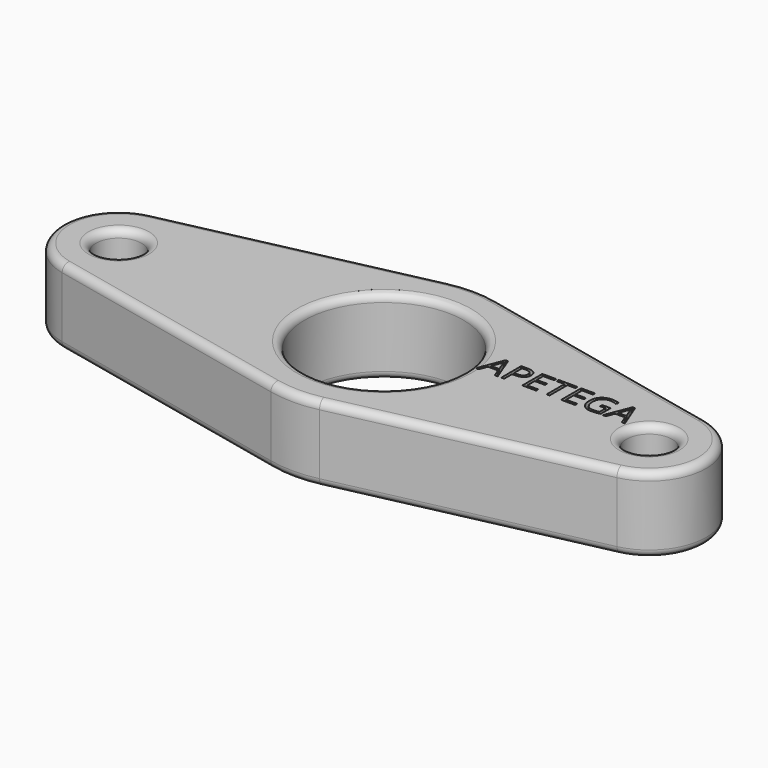
from build123d import *

# Parameters (mm, degrees)
F0_R         = 3
F0_R_2       = 10.5
F1_DEPTH     = 10
F2_R         = 1
F3_R         = 1
F4_TEXT_SIZE = 4.6232753016
F5_DEPTH     = 5


# Not quite as in the source:
# - Text() gives the source's letters only with a copy of the font that has no kerning and outlines rounded to 1/6400 em; it was checked with that copy


with BuildPart() as f1:
    # F0 (on Top) → F1 (new body)
    with BuildSketch(Plane.XY):
        with BuildLine():
            Line((-36.6071428571, -7.3257826774), (-3.2142857143, -14.6515653548))
            ThreePointArc((-3.2142857143, -14.6515653548), (0, -15), (3.2142857143, -14.6515653548))
            Line((3.2142857143, -14.6515653548), (36.6071428571, -7.3257826774))
            ThreePointArc((36.6071428571, -7.3257826774), (42.5, 0), (36.6071428571, 7.3257826774))
            Line((36.6071428571, 7.3257826774), (3.2142857143, 14.6515653548))
            ThreePointArc((3.2142857143, 14.6515653548), (0, 15), (-3.2142857143, 14.6515653548))
            Line((-3.2142857143, 14.6515653548), (-36.6071428571, 7.3257826774))
            ThreePointArc((-36.6071428571, 7.3257826774), (-42.5, 0), (-36.6071428571, -7.3257826774))
        make_face()
        with Locations((-35, 0)):
            Circle(F0_R, mode=Mode.SUBTRACT)
        Circle(F0_R_2, mode=Mode.SUBTRACT)
        with Locations((35, 0)):
            Circle(F0_R, mode=Mode.SUBTRACT)
    extrude(amount=F1_DEPTH)

    # F2
    f2_edges = [f1.edges().sort_by_distance(p)[0] for p in [
        (-19.910714, -10.988674, 10),
        (0, -15, 10),
        (19.910714, -10.988674, 10),
        (42.5, 0, 10),
        (19.910714, 10.988674, 10),
        (0, 15, 10),
        (-19.910714, 10.988674, 10),
        (-42.5, 0, 10),
        (-38, 0, 10),
        (-10.5, 0, 10),
        (32, 0, 10),
    ]]
    fillet(f2_edges, radius=F2_R)

    # F3
    f3_edges = [f1.edges().sort_by_distance(p)[0] for p in [
        (-19.910714, -10.988674, 0),
        (0, -15, 0),
        (19.910714, -10.988674, 0),
        (42.5, 0, 0),
        (19.910714, 10.988674, 0),
        (0, 15, 0),
        (-19.910714, 10.988674, 0),
        (-42.5, 0, 0),
        (-38, 0, 0),
        (-10.5, 0, 0),
        (32, 0, 0),
    ]]
    fillet(f3_edges, radius=F3_R)

    # F4 (on face) → F5 (cut)
    with BuildSketch(Plane.XY.offset(10)):
        with Locations((11.1675286724, 1.1454970639)):
            Text('APETEGA', F4_TEXT_SIZE, font='Open Sans', text_align=(TextAlign.LEFT, TextAlign.BOTTOM))
    extrude(amount=-F5_DEPTH, mode=Mode.SUBTRACT)


solid = f1.part
